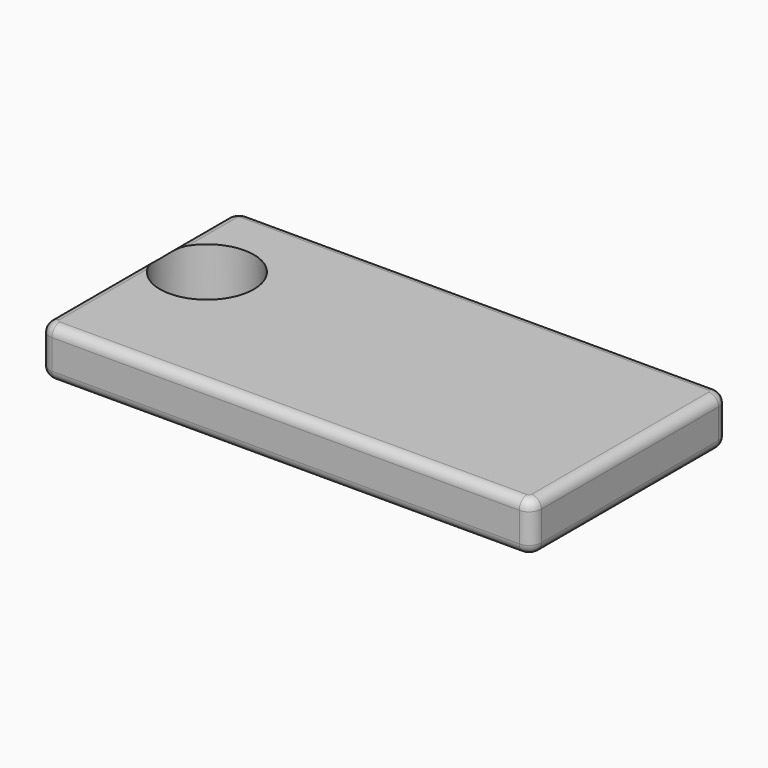
from build123d import *

# Parameters (mm, degrees)
F1_DEPTH     = 25.4
F2_R         = 24.2182856507
F3_DEPTH     = 25.401
F5_T1_DEPTH  = 114.3
F5_T3_DEPTH  = 241.3
F5_T6_ANGLE  = 90
F5_T8_ANGLE  = 90
F5_T10_ANGLE = 90
F5_T12_ANGLE = 90
F5_T14_ANGLE = 90
F5_T16_ANGLE = 90
F5_T18_ANGLE = 90
F5_T20_ANGLE = 90


# Not quite as in the source:
# - a fillet or chamfer that OpenCascade refuses, or shapes differently, is made with other operations: its cross-section is extruded or revolved along the edge and cut away or added
# - a feature of the source that left no trace in its solid (it failed there, or was rolled back) is left out


with BuildPart() as f1:
    # F0 (on Top) → F1 (new body)
    with BuildSketch(Plane.XY):
        with BuildLine():
            Line((120.65, 63.5), (-120.65, 63.5))
            ThreePointArc((-120.65, 63.5), (-125.1401280605, 61.6401280605), (-127, 57.15))
            Line((-127, 57.15), (-127, -57.15))
            ThreePointArc((-127, -57.15), (-125.1401280605, -61.6401280605), (-120.65, -63.5))
            Line((-120.65, -63.5), (120.65, -63.5))
            ThreePointArc((120.65, -63.5), (125.1401280605, -61.6401280605), (127, -57.15))
            Line((127, -57.15), (127, 57.15))
            ThreePointArc((127, 57.15), (125.1401280605, 61.6401280605), (120.65, 63.5))
        make_face()
    extrude(amount=F1_DEPTH)

    # F2 (on face) → F3 (cut, through all)
    with BuildSketch(Plane.XY.offset(25.4)):
        with Locations((-101.6, 12.7)):
            Circle(F2_R)
    extrude(amount=-F3_DEPTH, mode=Mode.SUBTRACT)

    # F5: fillet of radius 5.08 on 16 edges, made by hand

    # F5_s2 → F5_t1 (cut)
    with BuildSketch(Plane.XZ.offset(-57.15)):
        with BuildLine():
            ThreePointArc((121.92, 0), (125.5121024484, 1.4878975516), (127, 5.08))
            Line((127, 5.08), (127, 0))
            Line((127, 0), (121.92, 0))
        make_face()
        with BuildLine():
            ThreePointArc((-121.92, 0), (-125.5121024484, 1.4878975516), (-127, 5.08))
            Line((-127, 5.08), (-127, 0))
            Line((-127, 0), (-121.92, 0))
        make_face()
        with BuildLine():
            ThreePointArc((121.92, 25.4), (125.5121024484, 23.9121024484), (127, 20.32))
            Line((127, 20.32), (127, 25.4))
            Line((127, 25.4), (121.92, 25.4))
        make_face()
        with BuildLine():
            ThreePointArc((-121.92, 25.4), (-125.5121024484, 23.9121024484), (-127, 20.32))
            Line((-127, 20.32), (-127, 25.4))
            Line((-127, 25.4), (-121.92, 25.4))
        make_face()
    extrude(amount=F5_T1_DEPTH, mode=Mode.SUBTRACT)

    # F5_s4 → F5_t3 (cut)
    with BuildSketch(Plane.YZ.offset(-120.65)):
        with BuildLine():
            ThreePointArc((63.5, 5.08), (62.0121024484, 1.4878975516), (58.42, 0))
            Line((58.42, 0), (63.5, 0))
            Line((63.5, 0), (63.5, 5.08))
        make_face()
        with BuildLine():
            ThreePointArc((63.5, 20.32), (62.0121024484, 23.9121024484), (58.42, 25.4))
            Line((58.42, 25.4), (63.5, 25.4))
            Line((63.5, 25.4), (63.5, 20.32))
        make_face()
        with BuildLine():
            ThreePointArc((-58.42, 0), (-62.0121024484, 1.4878975516), (-63.5, 5.08))
            Line((-63.5, 5.08), (-63.5, 0))
            Line((-63.5, 0), (-58.42, 0))
        make_face()
        with BuildLine():
            ThreePointArc((-58.42, 25.4), (-62.0121024484, 23.9121024484), (-63.5, 20.32))
            Line((-63.5, 20.32), (-63.5, 25.4))
            Line((-63.5, 25.4), (-58.42, 25.4))
        make_face()
    extrude(amount=F5_T3_DEPTH, mode=Mode.SUBTRACT)

    # F5_s5 → F5_t6 (revolve, cut)
    with BuildSketch(Plane.XZ.offset(-57.15)):
        with BuildLine():
            ThreePointArc((127, 5.08), (125.5121024484, 1.4878975516), (121.92, 0))
            Line((121.92, 0), (127, 0))
            Line((127, 0), (127, 5.08))
        make_face()
    revolve(axis=Axis((120.65, 57.15, 0), (0, 0, 1)), revolution_arc=F5_T6_ANGLE, mode=Mode.SUBTRACT)

    # F5_s7 → F5_t8 (revolve, cut)
    with BuildSketch(Plane.XZ.offset(-57.15)):
        with BuildLine():
            ThreePointArc((127, 20.32), (125.5121024484, 23.9121024484), (121.92, 25.4))
            Line((121.92, 25.4), (127, 25.4))
            Line((127, 25.4), (127, 20.32))
        make_face()
    revolve(axis=Axis((120.65, 57.15, 25.4), (0, 0, 1)), revolution_arc=F5_T8_ANGLE, mode=Mode.SUBTRACT)

    # F5_s9 → F5_t10 (revolve, cut)
    with BuildSketch(Plane.YZ.offset(-120.65)):
        with BuildLine():
            ThreePointArc((63.5, 5.08), (62.0121024484, 1.4878975516), (58.42, 0))
            Line((58.42, 0), (63.5, 0))
            Line((63.5, 0), (63.5, 5.08))
        make_face()
    revolve(axis=Axis((-120.65, 57.15, 0), (0, 0, 1)), revolution_arc=F5_T10_ANGLE, mode=Mode.SUBTRACT)

    # F5_s11 → F5_t12 (revolve, cut)
    with BuildSketch(Plane.YZ.offset(-120.65)):
        with BuildLine():
            ThreePointArc((63.5, 20.32), (62.0121024484, 23.9121024484), (58.42, 25.4))
            Line((58.42, 25.4), (63.5, 25.4))
            Line((63.5, 25.4), (63.5, 20.32))
        make_face()
    revolve(axis=Axis((-120.65, 57.15, 25.4), (0, 0, 1)), revolution_arc=F5_T12_ANGLE, mode=Mode.SUBTRACT)

    # F5_s13 → F5_t14 (revolve, cut)
    with BuildSketch(Plane.YZ.offset(120.65)):
        with BuildLine():
            ThreePointArc((-58.42, 0), (-62.0121024484, 1.4878975516), (-63.5, 5.08))
            Line((-63.5, 5.08), (-63.5, 0))
            Line((-63.5, 0), (-58.42, 0))
        make_face()
    revolve(axis=Axis((120.65, -57.15, 0), (0, 0, 1)), revolution_arc=F5_T14_ANGLE, mode=Mode.SUBTRACT)

    # F5_s15 → F5_t16 (revolve, cut)
    with BuildSketch(Plane.XZ.offset(57.15)):
        with BuildLine():
            ThreePointArc((-121.92, 0), (-125.5121024484, 1.4878975516), (-127, 5.08))
            Line((-127, 5.08), (-127, 0))
            Line((-127, 0), (-121.92, 0))
        make_face()
    revolve(axis=Axis((-120.65, -57.15, 0), (0, 0, 1)), revolution_arc=F5_T16_ANGLE, mode=Mode.SUBTRACT)

    # F5_s17 → F5_t18 (revolve, cut)
    with BuildSketch(Plane.YZ.offset(120.65)):
        with BuildLine():
            ThreePointArc((-58.42, 25.4), (-62.0121024484, 23.9121024484), (-63.5, 20.32))
            Line((-63.5, 20.32), (-63.5, 25.4))
            Line((-63.5, 25.4), (-58.42, 25.4))
        make_face()
    revolve(axis=Axis((120.65, -57.15, 25.4), (0, 0, 1)), revolution_arc=F5_T18_ANGLE, mode=Mode.SUBTRACT)

    # F5_s19 → F5_t20 (revolve, cut)
    with BuildSketch(Plane.XZ.offset(57.15)):
        with BuildLine():
            ThreePointArc((-121.92, 25.4), (-125.5121024484, 23.9121024484), (-127, 20.32))
            Line((-127, 20.32), (-127, 25.4))
            Line((-127, 25.4), (-121.92, 25.4))
        make_face()
    revolve(axis=Axis((-120.65, -57.15, 25.4), (0, 0, 1)), revolution_arc=F5_T20_ANGLE, mode=Mode.SUBTRACT)


solid = f1.part
